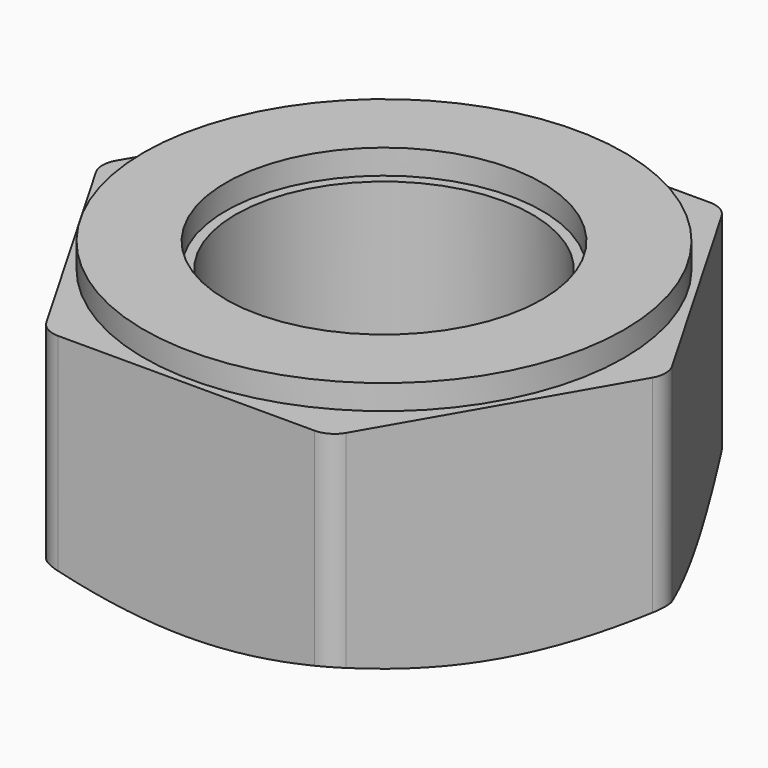
from build123d import *

# Parameters (mm, degrees)
F1_DEPTH    = 5
F4_R        = 3
F5_DEPTH    = 5.001
F6_R        = 0.5
F7_T1_DEPTH = 5.5598599904
F9_R        = 4.8595532258
F9_R_2      = 3.1997304912
F10_DEPTH   = 0.5


# Not quite as in the source:
# - a fillet or chamfer that OpenCascade refuses, or shapes differently, is made with other operations: its cross-section is extruded or revolved along the edge and cut away or added


with BuildPart() as f1:
    # F0 (on Top) → F1 (new body)
    with BuildSketch(Plane.XY):
        Polygon((-2.8867513459, 5), (-5.7735026919, 0), (-2.8867513459, -5), (2.8867513459, -5), (5.7735026919, 0), (2.8867513459, 5), align=None)
    extrude(amount=F1_DEPTH)

    # F2 (on Front) → F3 (revolve, cut)
    with BuildSketch(Plane.XZ):
        Polygon((6, 1), (3.5, -0.285714148), (6, -0.285714148), align=None)
    revolve(axis=Axis((0, 0, 1.7616122495), (0, 0, 1)), mode=Mode.SUBTRACT)

    # F4 (on face) → F5 (cut, through all)
    with BuildSketch(Plane(origin=(0, 0, 0), x_dir=(1, 0, 0), z_dir=(0, 0, -1))):
        Circle(F4_R)
    extrude(amount=-F5_DEPTH, mode=Mode.SUBTRACT)

    # F6
    f6_edges = [f1.edges().sort_by_distance(p)[0] for p in [
        (-2.886751, 5, 2.941758),
    ]]
    fillet(f6_edges, radius=F6_R)

    # F7: fillet of radius 0.5 on 5 edges, made by hand

    # F7_s2 → F7_t1 (cut)
    with BuildSketch(Plane.XY.offset(0.1618278461)):
        with BuildLine():
            ThreePointArc((-5.6291651246, 0.25), (-5.6961524227, 0), (-5.6291651246, -0.25))
            Line((-5.6291651246, -0.25), (-5.7735026919, 0))
            Line((-5.7735026919, 0), (-5.6291651246, 0.25))
        make_face()
        with BuildLine():
            ThreePointArc((-3.0310889132, -4.75), (-2.8480762114, -4.9330127019), (-2.5980762114, -5))
            Line((-2.5980762114, -5), (-2.8867513459, -5))
            Line((-2.8867513459, -5), (-3.0310889132, -4.75))
        make_face()
        with BuildLine():
            ThreePointArc((2.5980762114, -5), (2.8480762114, -4.9330127019), (3.0310889132, -4.75))
            Line((3.0310889132, -4.75), (2.8867513459, -5))
            Line((2.8867513459, -5), (2.5980762114, -5))
        make_face()
        with BuildLine():
            ThreePointArc((5.6291651246, 0.25), (5.6961524227, 0), (5.6291651246, -0.25))
            Line((5.6291651246, -0.25), (5.7735026919, 0))
            Line((5.7735026919, 0), (5.6291651246, 0.25))
        make_face()
        with BuildLine():
            ThreePointArc((2.5980762114, 5), (2.8480762114, 4.9330127019), (3.0310889132, 4.75))
            Line((3.0310889132, 4.75), (2.8867513459, 5))
            Line((2.8867513459, 5), (2.5980762114, 5))
        make_face()
    extrude(amount=F7_T1_DEPTH, mode=Mode.SUBTRACT)

    # F9 (on face) → F10 (join)
    with BuildSketch(Plane.XY.offset(5)):
        Circle(F9_R)
        Circle(F9_R_2, mode=Mode.SUBTRACT)
    extrude(amount=F10_DEPTH)


solid = f1.part
